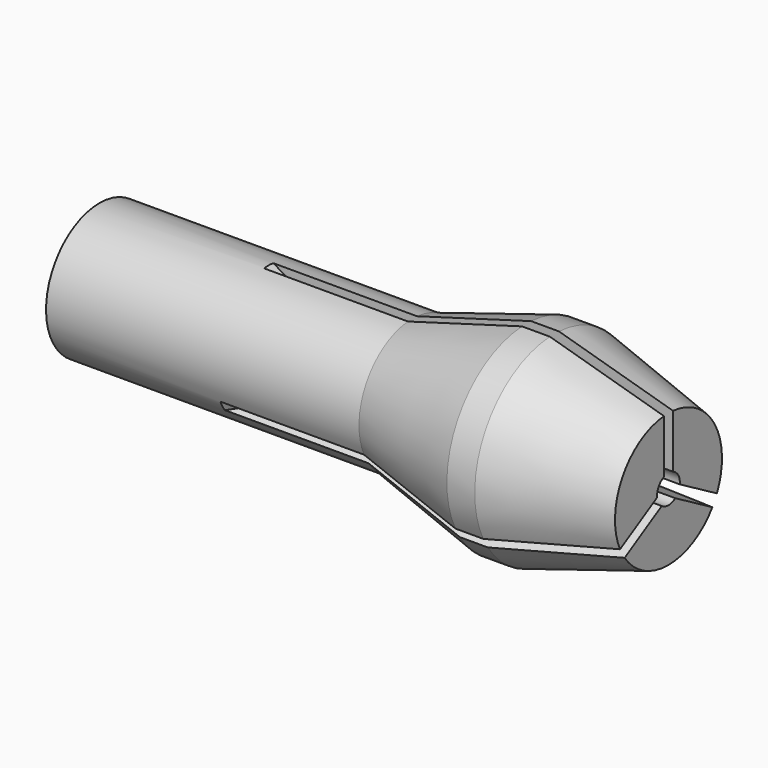
from build123d import *

# Parameters (mm, degrees)
F3_DEPTH        = 0.2
F3_COPIES_COUNT = 3


# Not quite as in the source:
# - a pattern or mirror of a feature is missing from the dataset's text; its kind, count and spacing are read off the source's solid


with BuildPart() as f1:
    # F0 (on Front) → F1 (revolve)
    with BuildSketch(Plane.XZ):
        Polygon((0, 2.35), (0, 1), (12, 1), (12.3004303095, 0.5), (20, 0.5), (20, 2.35), (15.9894733896, 3.5), (15.0105266104, 3.5), (11, 2.35), align=None)
    revolve(axis=Axis((16.0586256534, 0, 0), (1, 0, 0)))

    # F2 (on Front) → F3 (cut, symmetric)
    with BuildSketch(Plane.XZ):
        with BuildLine():
            Line((14, 15), (14, 0.5))
            Line((14, 0.5), (17.8405728739, 0.5))
            ThreePointArc((17.8405728739, 0.5), (25.8871483777, 5.8514644098), (29, 15))
            Line((29, 15), (14, 15))
        make_face()
        with BuildLine():
            Line((14, 0), (14, 0.5))
            Line((14, 0.5), (14, 15))
            Line((14, 15), (29, 15))
            ThreePointArc((29, 15), (6.7858795946, 28.151291449), (5.9391377632, 2.35))
            ThreePointArc((5.9391377632, 2.35), (7.2431859715, 1.6080074603), (8.6148351929, 1))
            ThreePointArc((8.6148351929, 1), (11.2613872125, 0.2521187962), (14, 0))
        make_face()
        with BuildLine():
            Line((17.8405728739, 0.5), (14, 0.5))
            Line((14, 0.5), (14, 0))
            ThreePointArc((14, 0), (15.9364916731, 0.1255252194), (17.8405728739, 0.5))
        make_face()
        with BuildLine():
            ThreePointArc((29, 15), (25.8871483777, 5.8514644098), (17.8405728739, 0.5))
            ThreePointArc((17.8405728739, 0.5), (15.9364916731, 0.1255252194), (14, 0))
            Line((14, 0), (29, 0))
            Line((29, 0), (29, 15))
        make_face()
    f3 = extrude(amount=F3_DEPTH, both=True, mode=Mode.SUBTRACT)

    # F3_copies: F3 ×3 about axis
    f3_copies_axis = Axis((0, 0, 0), (1, 0, 0))
    for i in range(1, F3_COPIES_COUNT):
        add(f3.rotate(f3_copies_axis, i * 360 / F3_COPIES_COUNT), mode=Mode.SUBTRACT)


solid = f1.part
